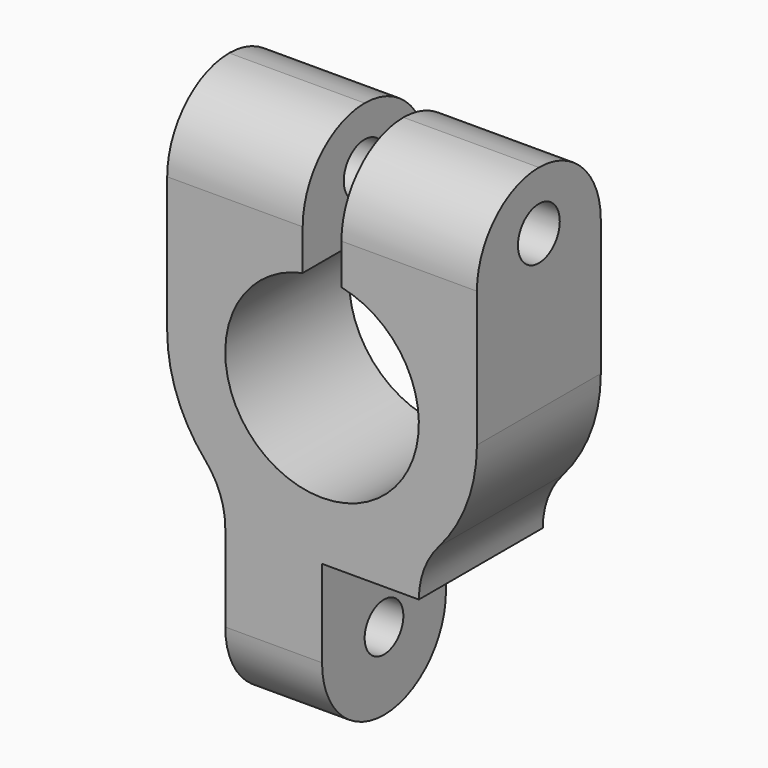
from build123d import *

# Parameters (mm, degrees)
F1_DEPTH = 4
F2_R     = 1.35
F3_DEPTH = 25
F4_R     = 1.25
F5_DEPTH = 25
F6_R     = 3.99999


# Not quite as in the source:
# - a fillet or chamfer is up to 0.001 mm smaller than in the source, because OpenCascade refuses the exact size
# - a feature names something its author has since deleted; it is built from what else it names


with BuildPart() as f1:
    # F0 (on Front) → F1 (new body, symmetric)
    with BuildSketch(Plane.XZ):
        with BuildLine():
            ThreePointArc((1, 4.8989794856), (0, -5), (-1, 4.8989794856))
            Line((-1, 4.8989794856), (-1, 11))
            Line((-1, 11), (-8, 11))
            Line((-8, 11), (-8, 0))
            ThreePointArc((-8, 0), (-7.4906334206, -2.8089875327), (-6.0273972603, -5.2602739726))
            ThreePointArc((-6.0273972603, -5.2602739726), (-5.2652950935, -6.53698566), (-5, -8))
            Line((-5, -8), (-5, -16.5))
            Line((-5, -16.5), (0, -16.5))
            Line((0, -16.5), (0, -8))
            Line((0, -8), (5, -8))
            ThreePointArc((5, -8), (5.2652950935, -6.53698566), (6.0273972603, -5.2602739726))
            ThreePointArc((6.0273972603, -5.2602739726), (7.4906334206, -2.8089875327), (8, 0))
            Line((8, 0), (8, 11))
            Line((8, 11), (1, 11))
            Line((1, 11), (1, 4.8989794856))
        make_face()
    extrude(amount=F1_DEPTH, both=True)

    # F2 (on face) → F3 (cut)
    with BuildSketch(Plane.YZ.offset(8)):
        with Locations((0, 8)):
            Circle(F2_R)
    extrude(amount=-F3_DEPTH, mode=Mode.SUBTRACT)

    # F4 (on face) → F5 (cut)
    with BuildSketch(Plane.YZ):
        with Locations((0, -12.5)):
            Circle(F4_R)
    extrude(amount=-F5_DEPTH, mode=Mode.SUBTRACT)

    # F6 (radius 4 in the source; OpenCascade refuses exactly that, so slightly less here)
    f6_edges = [f1.edges().sort_by_distance(p)[0] for p in [
        (-4.5, -4, 11),
        (-4.5, 4, 11),
        (4.5, 4, 11),
        (-2.5, -4, -16.5),
        (-2.5, 4, -16.5),
        (4.5, -4, 11),
    ]]
    fillet(f6_edges, radius=F6_R)


solid = f1.part
